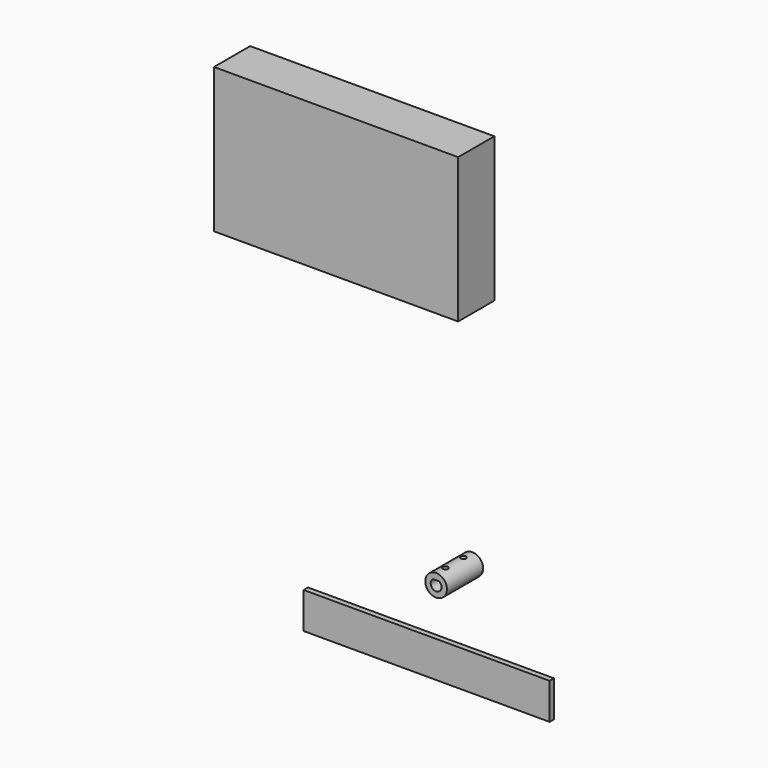
from build123d import *

# Parameters (mm, degrees)
F0_R      = 6
F1_DEPTH  = 25
F2_R      = 3
F3_DEPTH  = 25
F5_DEPTH  = 25
F6_R      = 1.5
F7_DEPTH  = 3.5
F8_W      = 136
F8_H      = 20
F9_DEPTH  = 3
F11_W     = 135
F11_H     = 80
F12_DEPTH = 25


with BuildPart() as f1:
    # F0 (on Front) → F1 (new body)
    with BuildSketch(Plane.XZ):
        Circle(F0_R)
    extrude(amount=F1_DEPTH)

    # F2 (on Front) → F3 (cut, through all)
    with BuildSketch(Plane.XZ):
        Circle(F2_R)
    extrude(amount=F3_DEPTH, mode=Mode.SUBTRACT)

    # F4 (on face) → F5 (join, through all)
    with BuildSketch(Plane.XZ.offset(25)):
        with BuildLine():
            Line((-1.6583123952, 2.5), (0, 2.5))
            Line((0, 2.5), (1.6583123952, 2.5))
            ThreePointArc((1.6583123952, 2.5), (0, 3), (-1.6583123952, 2.5))
        make_face()
    extrude(amount=-F5_DEPTH)

    # F6 (on face) → F7 (cut, through all)
    with BuildSketch(Plane(origin=(0, 0, 2.5), x_dir=(1, 0, 0), z_dir=(0, 0, -1))):
        with Locations((0, 18.75)):
            Circle(F6_R)
        with Locations((0, 6.25)):
            Circle(F6_R)
    extrude(amount=-F7_DEPTH, mode=Mode.SUBTRACT)


with BuildPart() as f9:
    # F8 (on face) → F9 (new body)
    with BuildSketch(Plane.XZ.offset(25)):
        with Locations((-2.8303451836, -34.0883203877)):
            Rectangle(F8_W, F8_H)
    extrude(amount=F9_DEPTH)


with BuildPart() as f12:
    # F11 (on face) → F12 (new body)
    with BuildSketch(Plane.XZ.offset(28)):
        with Locations((-32.9120505211, 191.017486155)):
            Rectangle(F11_W, F11_H)
    extrude(amount=F12_DEPTH)


solid = Compound([f1.part, f9.part, f12.part])
